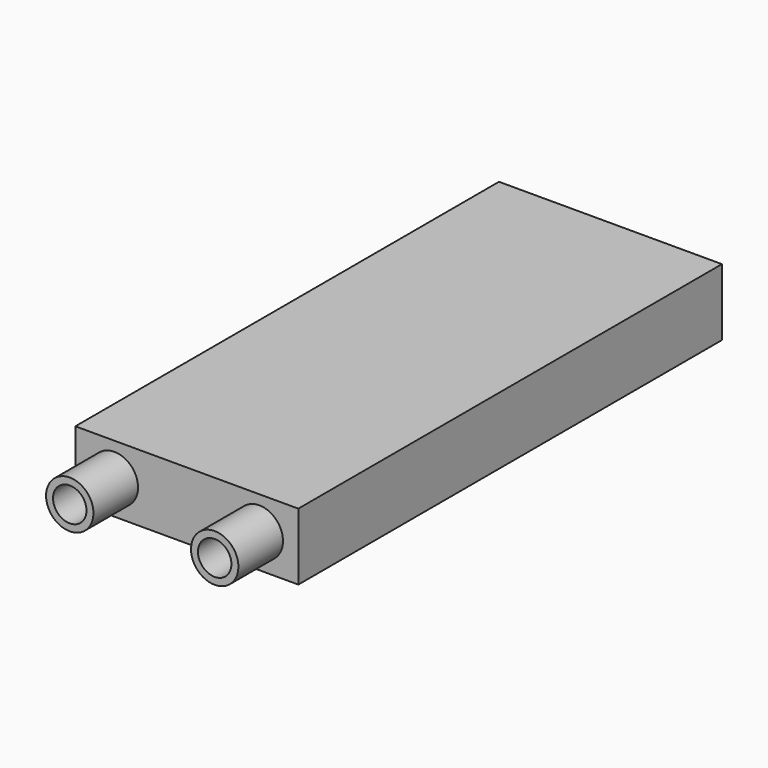
from build123d import *

# Parameters (mm, degrees)
F0_W     = 20
F0_H     = 95
F1_DEPTH = 6
F3_R     = 3
F5_R     = 4.25
F5_R_2   = 3
F6_DEPTH = 10


with BuildPart() as f1:
    # F0 (on Top) → F1 (new body, symmetric)
    with BuildSketch(Plane.XY):
        with Locations((10, 47.5)):
            Rectangle(F0_W, F0_H)
    extrude(amount=F1_DEPTH, both=True)

    # F4: sweep along a path in F2
    with BuildLine(Plane.XY) as f4_path:
        Line((13, 0), (13, 80))
        ThreePointArc((13, 80), (10.6568542495, 85.6568542495), (5, 88))
        Line((5, 88), (0, 88))
    # F3 (on face) → F4 (sweep, cut)
    with BuildSketch(Plane.XZ):
        with Locations((13, 0)):
            Circle(F3_R)
    sweep(path=f4_path.line, mode=Mode.SUBTRACT)

    # F5 (on face) → F6 (join)
    with BuildSketch(Plane.XZ):
        with Locations((13, 0)):
            Circle(F5_R)
        with Locations((13, 0)):
            Circle(F5_R_2, mode=Mode.SUBTRACT)
    extrude(amount=F6_DEPTH)

    # F7: F1 across face


with BuildPart() as f1_1:
    add(f1.part)
    add(f1.part.mirror(Plane(origin=(0, 46.4699702389, 0), x_dir=(0, -1, 0), z_dir=(-1, 0, 0))))


solid = f1_1.part
